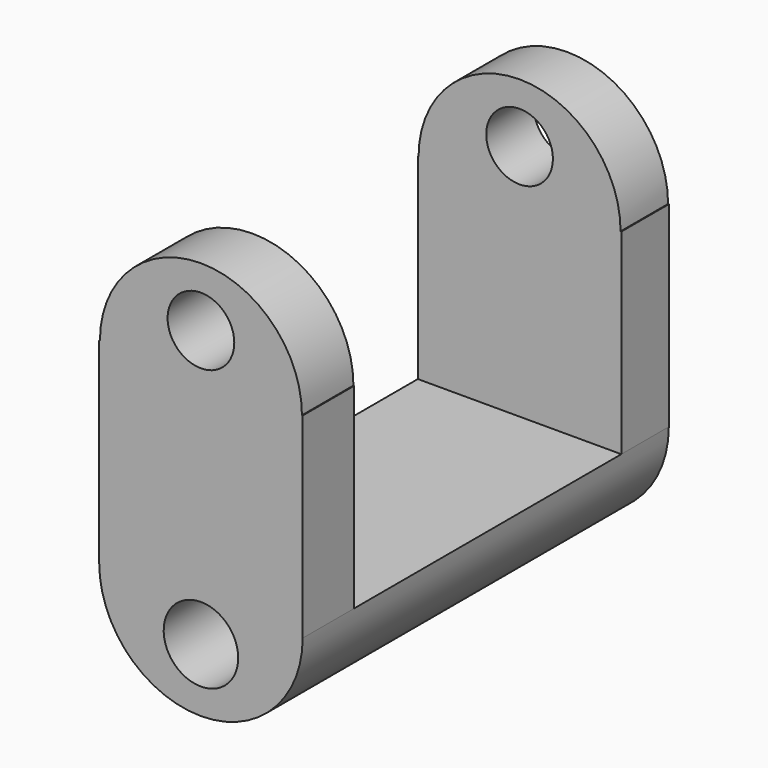
from build123d import *

# Parameters (mm, degrees)
F0_R          = 7.3981618973
F1_DEPTH      = 50.8
F1_DEPTH_BACK = 50.8
F2_W          = 74.1309896111
F2_H          = 66.0332143307
F3_DEPTH      = 25.4
F3_DEPTH_BACK = 25.4


# Not quite as in the source:
# - the program builds the solid bodies; features that only make, move or delete a surface that nothing else refers to are left out


with BuildPart() as f1:
    # F0 (on Front) → F1 (new body, two sides)
    with BuildSketch(Plane.XZ) as f1_sk:
        with BuildLine():
            Line((-22.5902460515, 0), (-22.5853170946, 0))
            ThreePointArc((-22.5853170946, 0), (0, -22.5853170946), (22.5853170946, 0))
            Line((22.5853170946, 0), (22.5902460515, 0))
            Line((22.5902460515, 0), (22.5902460515, 43.5050576925))
            Line((22.5902460515, 43.5050576925), (22.4241250182, 43.5050576925))
            ThreePointArc((22.4241250182, 43.5050576925), (0, 65.9291827108), (-22.4241250182, 43.5050576925))
            Line((-22.4241250182, 43.5050576925), (-22.5902460515, 43.5050576925))
            Line((-22.5902460515, 43.5050576925), (-22.5902460515, 0))
        make_face()
        with BuildLine():
            ThreePointArc((0, -0.2681852946), (5.848754541, -2.6908187485), (8.2713879948, -8.5395732895))
            ThreePointArc((8.2713879948, -8.5395732895), (-5.848754541, -14.3883278304), (0, -0.2681852946))
        make_face(mode=Mode.SUBTRACT)
        with Locations((0, 52.7734495699)):
            Circle(F0_R, mode=Mode.SUBTRACT)
    extrude(amount=F1_DEPTH)
    extrude(f1_sk.sketch, amount=-F1_DEPTH_BACK)

    # F2 (on Right) → F3 (cut, two sides)
    with BuildSketch(Plane.YZ) as f3_sk:
        with Locations((0.5546920002, 33.0166071653)):
            Rectangle(F2_W, F2_H)
    extrude(amount=-F3_DEPTH, mode=Mode.SUBTRACT)
    extrude(f3_sk.sketch, amount=F3_DEPTH_BACK, mode=Mode.SUBTRACT)


solid = f1.part
